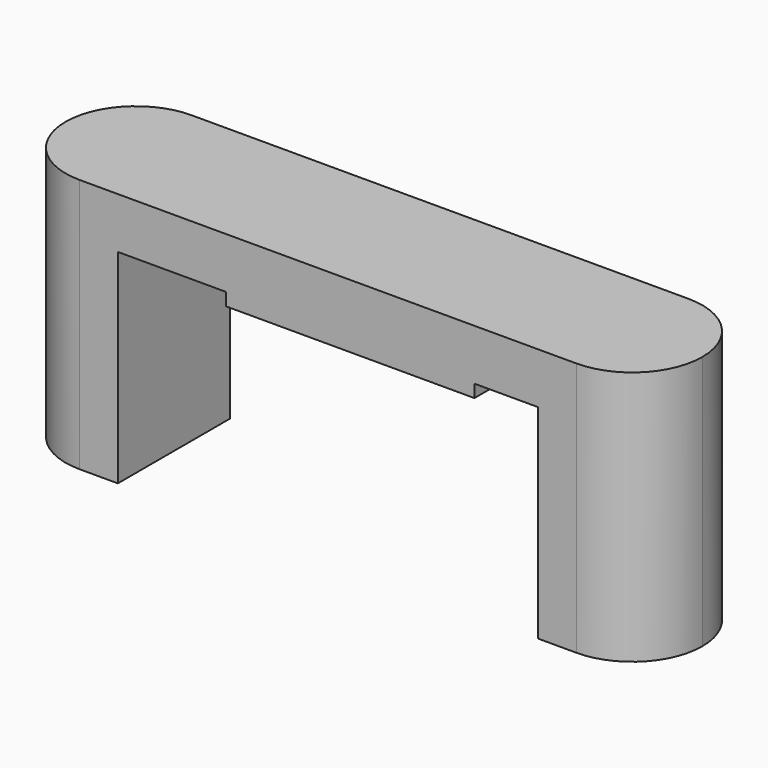
from build123d import *

# Parameters (mm, degrees)
F1_DEPTH = 5.5
F2_R     = 1.125
F3_DEPTH = 4
F4_R     = 2.74999


# Not quite as in the source:
# - a fillet or chamfer is up to 0.001 mm smaller than in the source, because OpenCascade refuses the exact size


with BuildPart() as f1:
    # F0 (on Front) → F1 (new body)
    with BuildSketch(Plane.XZ):
        Polygon((-12.5, 10), (-12.5, 0), (-8.25, 0), (-8.25, 8), (-4, 8), (-4, 7.5), (5.75, 7.5), (5.75, 8), (8.25, 8), (8.25, 0), (12.5, 0), (12.5, 10), align=None)
    extrude(amount=F1_DEPTH)

    # F2 (on face) → F3 (cut)
    with BuildSketch(Plane(origin=(0, 0, 0), x_dir=(1, 0, 0), z_dir=(0, 0, -1))):
        with Locations((-9.75, 2.75)):
            Circle(F2_R)
        with Locations((9.75, 2.75)):
            Circle(F2_R)
    extrude(amount=-F3_DEPTH, mode=Mode.SUBTRACT)

    # F4 (radius 2.75 in the source; OpenCascade refuses exactly that, so slightly less here)
    f4_edges = [f1.edges().sort_by_distance(p)[0] for p in [
        (-12.5, -5.5, 5),
        (-12.5, 0, 5),
        (12.5, -5.5, 5),
        (12.5, 0, 5),
    ]]
    fillet(f4_edges, radius=F4_R)


solid = f1.part
